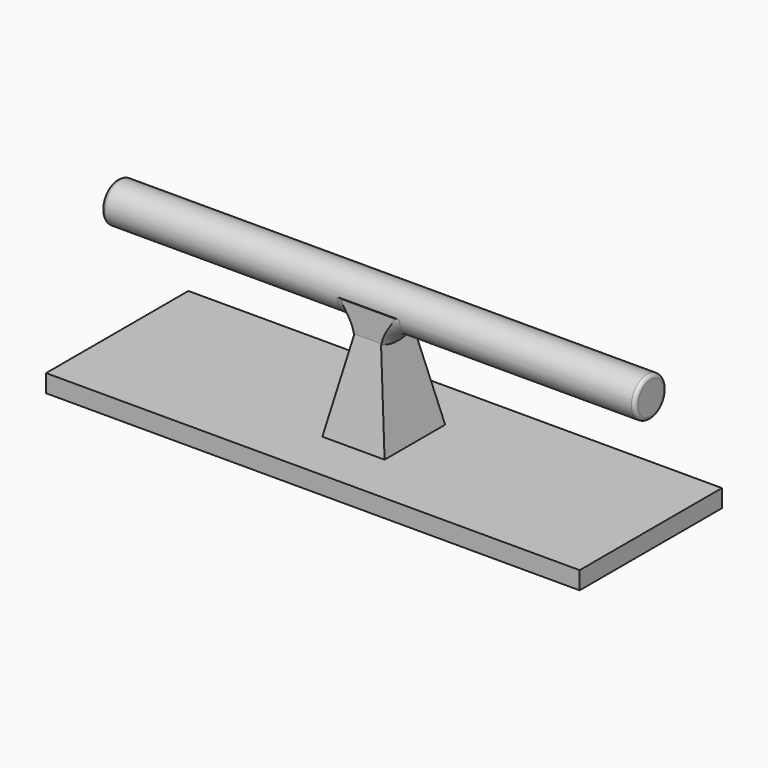
from build123d import *

# Parameters (mm, degrees)
F0_R         = 11.1
F1_DEPTH     = 150
F2_W         = 22.5644709975
F2_H         = 75
F4_DEPTH     = 7.5
F5_W         = 300
F5_H         = 100
F5_W_2       = 15
F5_H_2       = 22.5644709975
F7_DEPTH     = 10
F8_SIZE2     = 50
F8_SIZE      = 10
F9_T4_ANGLE  = 180
F9_T10_ANGLE = 180


# Not quite as in the source:
# - a fillet or chamfer that OpenCascade refuses, or shapes differently, is made with other operations: its cross-section is extruded or revolved along the edge and cut away or added


with BuildPart() as f1:
    # F0 (on Right) → F1 (new body, symmetric)
    with BuildSketch(Plane.YZ):
        Circle(F0_R)
    extrude(amount=F1_DEPTH, both=True)

    # F2 (on Right) → F4 (join, symmetric)
    with BuildSketch(Plane.YZ):
        with Locations((-0.1822354987, -37.5)):
            Rectangle(F2_W, F2_H)
    extrude(amount=F4_DEPTH, both=True)

    # F6: fillet of radius 2 on 2 edges, made by hand

    # F6_s1 → F6_t2 (revolve, cut)
    with BuildSketch(Plane.XY):
        with BuildLine():
            ThreePointArc((-148, 11.1), (-149.4142135624, 10.5142135624), (-150, 9.1))
            Line((-150, 9.1), (-150, 11.1))
            Line((-150, 11.1), (-148, 11.1))
        make_face()
    revolve(axis=Axis((-150, 0, 0), (1, 0, 0)), mode=Mode.SUBTRACT)

    # F6_s3 → F6_t4 (revolve, cut)
    with BuildSketch(Plane.XY):
        with BuildLine():
            ThreePointArc((148, 11.1), (149.4142135624, 10.5142135624), (150, 9.1))
            Line((150, 9.1), (150, 11.1))
            Line((150, 11.1), (148, 11.1))
        make_face()
    revolve(axis=Axis((150, 0, 0), (1, 0, 0)), mode=Mode.SUBTRACT)

    # F5 (on face) → F7 (join)
    with BuildSketch(Plane(origin=(0, 0, -75), x_dir=(1, 0, 0), z_dir=(0, 0, -1))):
        Rectangle(F5_W, F5_H)
        with Locations((0, 0.1822354987)):
            Rectangle(F5_W_2, F5_H_2, mode=Mode.SUBTRACT)
    extrude(amount=-F7_DEPTH)

    # F8
    f8_edges = [f1.edges().sort_by_distance(p)[0] for p in [
        (7.5, -0.182235, -65),
        (0, -11.464471, -65),
        (0, 11.1, -65),
        (-7.5, -0.182235, -65),
    ]]
    f8_side = f1.faces().sort_by_distance((146.837722, 0, -65))[0]
    chamfer(f8_edges, length=F8_SIZE, length2=F8_SIZE2, reference=f8_side)

    # F9: fillet of radius 10 on 2 edges, made by hand


with BuildPart() as f9_tool2:
    # F9_s3 → F9_t4 (revolve)
    with BuildSketch(Plane.XY):
        with BuildLine():
            ThreePointArc((7.5, -21.1), (10.4289321881, -14.0289321881), (17.5, -11.1))
            Line((17.5, -11.1), (7.5, -11.1))
            Line((7.5, -11.1), (7.5, -21.1))
        make_face()
    revolve(axis=Axis((7.5, 0, 0), (1, 0, 0)), revolution_arc=F9_T4_ANGLE)

    split(bisect_by=Plane.XZ.offset(-11.1), keep=Keep.TOP)

    split(bisect_by=Plane.XZ.offset(11.4644709975), keep=Keep.BOTTOM)


with BuildPart() as f1_1:
    add(f1.part)

    # F9_t1: union F9_tool2
    add(f9_tool2.part)


with BuildPart() as f9_tool8:
    # F9_s9 → F9_t10 (revolve)
    with BuildSketch(Plane.XY):
        with BuildLine():
            ThreePointArc((-17.5, -11.1), (-10.4289321881, -14.0289321881), (-7.5, -21.1))
            Line((-7.5, -21.1), (-7.5, -11.1))
            Line((-7.5, -11.1), (-17.5, -11.1))
        make_face()
    revolve(axis=Axis((-7.5, 0, 0), (1, 0, 0)), revolution_arc=F9_T10_ANGLE)

    split(bisect_by=Plane.XZ.offset(-11.1), keep=Keep.TOP)

    split(bisect_by=Plane.XZ.offset(11.4644709975), keep=Keep.BOTTOM)


with BuildPart() as f1_2:
    add(f1_1.part)

    # F9_t7: union F9_tool8
    add(f9_tool8.part)


solid = f1_2.part
